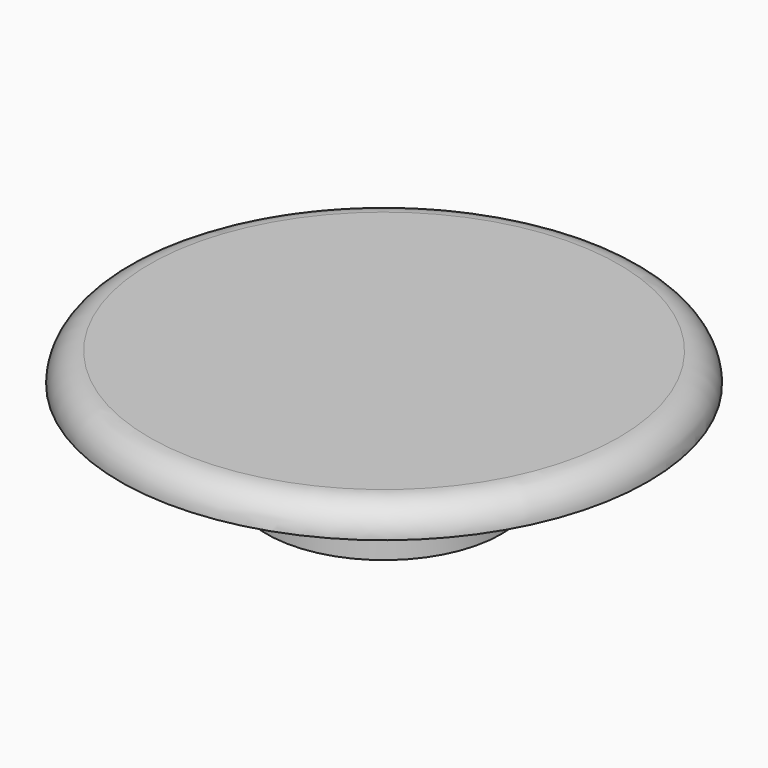
from build123d import *

# Parameters (mm, degrees)
F2_R = 0.99999


# Not quite as in the source:
# - a fillet or chamfer is up to 0.001 mm smaller than in the source, because OpenCascade refuses the exact size


with BuildPart() as f1:
    # F0 (on Front) → F1 (revolve)
    with BuildSketch(Plane.XZ):
        Polygon((0, 4.2), (0, 0), (4, 0), (4, 2), (5, 2), (5, 3.2), (9, 3.2), (9, 4.2), align=None)
    revolve(axis=Axis((0, 0, 2.1), (0, 0, -1)))

    # F2 (radius 1 in the source; OpenCascade refuses exactly that, so slightly less here)
    f2_edges = [f1.edges().sort_by_distance(p)[0] for p in [
        (-9, 0, 4.2),
    ]]
    fillet(f2_edges, radius=F2_R)


solid = f1.part
